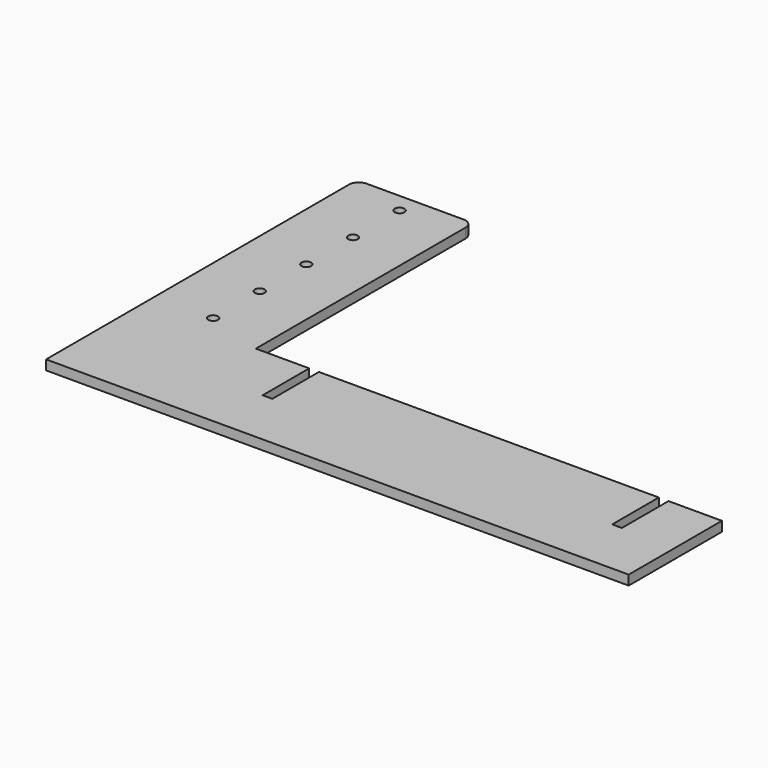
from build123d import *

# Parameters (mm, degrees)
F0_W     = 76.2
F0_H     = 76.2
F1_DEPTH = 6.35
F2_R     = 3.175
F3_DEPTH = 25.4


# Not quite as in the source:
# - a feature names something its author has since deleted; it is built from what else it names


with BuildPart() as f1:
    # F0 (on Top) → F1 (new body)
    with BuildSketch(Plane.XY):
        with BuildLine():
            Line((0, 0), (76.2, 0))
            Line((76.2, 0), (76.2, 171.45))
            ThreePointArc((76.2, 171.45), (74.3401280605, 175.9401280605), (69.85, 177.8))
            Line((69.85, 177.8), (6.35, 177.8))
            ThreePointArc((6.35, 177.8), (1.8598719395, 175.9401280605), (0, 171.45))
            Line((0, 171.45), (0, 0))
        make_face()
        with Locations((38.1, -38.1)):
            Rectangle(F0_W, F0_H)
        Polygon((111.125, -38.1), (111.125, 0), (76.2, 0), (76.2, -76.2), (250.825, -76.2), (257.175, -76.2), (381, -76.2), (381, 0), (346.075, 0), (346.075, -38.1), (342.9, -38.1), (339.725, -38.1), (339.725, 0), (257.175, 0), (250.825, 0), (117.475, 0), (117.475, -38.1), (114.3, -38.1), align=None)
    extrude(amount=F1_DEPTH)

    # F2 (on face) → F3 (cut)
    with BuildSketch(Plane.XY.offset(6.35)):
        with Locations((38.1, 12.7454660833)):
            Circle(F2_R)
        with Locations((38.1, 50.8454660833)):
            Circle(F2_R)
        with Locations((38.1, 88.9454660833)):
            Circle(F2_R)
        with Locations((38.1, 127.0454660833)):
            Circle(F2_R)
        with Locations((38.1, 165.1454660833)):
            Circle(F2_R)
    extrude(amount=-F3_DEPTH, mode=Mode.SUBTRACT)


solid = f1.part
